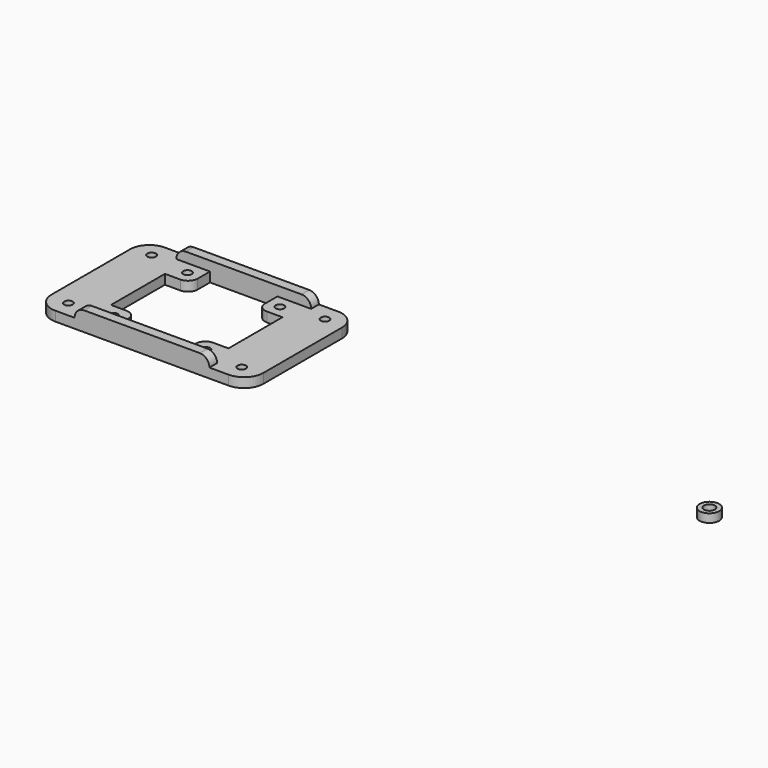
from build123d import *

# Parameters (mm, degrees)
F0_R     = 2.2
F1_DEPTH = 5
F2_R     = 10
F4_DEPTH = 5
F5_R     = 4.99999
F6_R     = 5.1
F6_R_2   = 2.85
F7_DEPTH = 4.4


# Not quite as in the source:
# - a fillet or chamfer is up to 0.001 mm smaller than in the source, because OpenCascade refuses the exact size


with BuildPart() as f1:
    # F0 (on Top) → F1 (new body)
    with BuildSketch(Plane.XY):
        Polygon((-207.6542276144, -31.5558707826), (-152.6542276144, -31.5558707826), (-97.6542276144, -31.5558707826), (-97.6542276144, 39.4441292174), (-152.6542276144, 39.4441292174), (-207.6542276144, 39.4441292174), align=None)
        with Locations((-197.6542276144, -23.0558707826)):
            Circle(F0_R, mode=Mode.SUBTRACT)
        with Locations((-176.6542276144, -20.0558707826)):
            Circle(F0_R, mode=Mode.SUBTRACT)
        with Locations((-128.6542276144, -20.0558707826)):
            Circle(F0_R, mode=Mode.SUBTRACT)
        with Locations((-107.6542276144, -23.0558707826)):
            Circle(F0_R, mode=Mode.SUBTRACT)
        with Locations((-197.6542276144, 30.9441292174)):
            Circle(F0_R, mode=Mode.SUBTRACT)
        with Locations((-176.6542276144, 27.9441292174)):
            Circle(F0_R, mode=Mode.SUBTRACT)
        with BuildLine():
            Line((-175.1542276144, -13.5558707826), (-183.1542276144, -13.5558707826))
            Line((-183.1542276144, -13.5558707826), (-183.1542276144, 21.4441292174))
            Line((-183.1542276144, 21.4441292174), (-175.1542276144, 21.4441292174))
            ThreePointArc((-175.1542276144, 21.4441292174), (-171.6186937085, 22.9085953115), (-170.1542276144, 26.4441292174))
            Line((-170.1542276144, 26.4441292174), (-170.1542276144, 34.4441292174))
            Line((-170.1542276144, 34.4441292174), (-135.1542276144, 34.4441292174))
            Line((-135.1542276144, 34.4441292174), (-135.1542276144, 25.4441292174))
            ThreePointArc((-135.1542276144, 25.4441292174), (-133.3785159981, 22.5387687378), (-130.1542276144, 21.4441292174))
            Line((-130.1542276144, 21.4441292174), (-122.1542276144, 21.4441292174))
            Line((-122.1542276144, 21.4441292174), (-122.1542276144, -13.5558707826))
            Line((-122.1542276144, -13.5558707826), (-130.1542276144, -13.5558707826))
            ThreePointArc((-130.1542276144, -13.5558707826), (-133.6897615203, -15.0203368767), (-135.1542276144, -18.5558707826))
            Line((-135.1542276144, -18.5558707826), (-135.1542276144, -26.5558707826))
            Line((-135.1542276144, -26.5558707826), (-170.1542276144, -26.5558707826))
            Line((-170.1542276144, -26.5558707826), (-170.1542276144, -18.5558707826))
            ThreePointArc((-170.1542276144, -18.5558707826), (-171.6186937085, -15.0203368767), (-175.1542276144, -13.5558707826))
        make_face(mode=Mode.SUBTRACT)
        with Locations((-128.6542276144, 27.9441292174)):
            Circle(F0_R, mode=Mode.SUBTRACT)
        with Locations((-107.6542276144, 30.9441292174)):
            Circle(F0_R, mode=Mode.SUBTRACT)
    extrude(amount=F1_DEPTH)

    # F2
    f2_edges = [f1.edges().sort_by_distance(p)[0] for p in [
        (-207.654228, -31.555871, 2.5),
        (-207.654228, 39.444129, 2.5),
        (-97.654228, -31.555871, 2.5),
        (-97.654228, 39.444129, 2.5),
    ]]
    fillet(f2_edges, radius=F2_R)

    # F3 (on face) → F4 (join)
    with BuildSketch(Plane.XY.offset(5)):
        Polygon((-117.6542276144, 34.4441292174), (-117.6542276144, 39.4441292174), (-187.6542276144, 39.4441292174), (-187.6542276144, 34.4441292174), (-170.1542276144, 34.4441292174), (-135.1542276144, 34.4441292174), align=None)
        Polygon((-117.6542276144, -26.5558707826), (-135.1542276144, -26.5558707826), (-170.1542276144, -26.5558707826), (-187.6542276144, -26.5558707826), (-187.6542276144, -31.5558707826), (-117.6542276144, -31.5558707826), align=None)
    extrude(amount=F4_DEPTH)

    # F5 (radius 5 in the source; OpenCascade refuses exactly that, so slightly less here)
    f5_edges = [f1.edges().sort_by_distance(p)[0] for p in [
        (-187.654228, -29.055871, 10),
        (-117.654228, -29.055871, 10),
        (-117.654228, 36.944129, 10),
        (-187.654228, 36.944129, 10),
    ]]
    fillet(f5_edges, radius=F5_R)


with BuildPart() as f7:
    # F6 (on Top) → F7 (new body)
    with BuildSketch(Plane.XY):
        with Locations((116.6157959732, 0)):
            Circle(F6_R)
        with Locations((116.6157959732, 0)):
            Circle(F6_R_2, mode=Mode.SUBTRACT)
    extrude(amount=F7_DEPTH)


solid = Compound([f1.part, f7.part])
